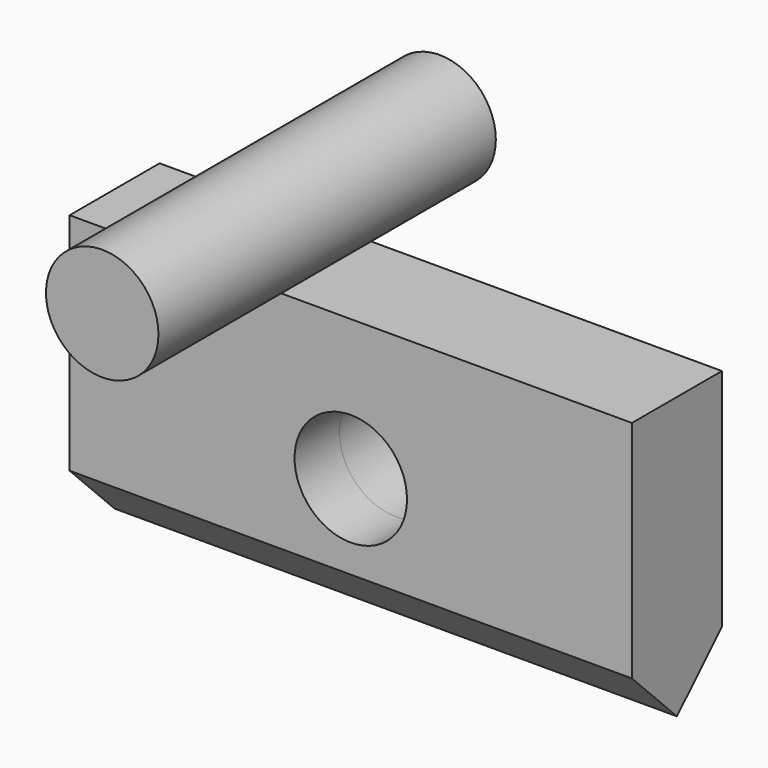
from build123d import *

# Parameters (mm, degrees)
F0_W          = 200
F0_H          = 100
F0_R          = 20
F1_DEPTH      = 20
F1_DEPTH_BACK = 20
F2_SIZE       = 19.99999
F3_R          = 20
F4_DEPTH      = 150


# Not quite as in the source:
# - a fillet or chamfer is up to 0.001 mm smaller than in the source, because OpenCascade refuses the exact size


with BuildPart() as f1:
    # F0 (on Front) → F1 (new body, two sides)
    with BuildSketch(Plane.XZ) as f1_sk:
        Rectangle(F0_W, F0_H)
        Circle(F0_R, mode=Mode.SUBTRACT)
    extrude(amount=F1_DEPTH)
    extrude(f1_sk.sketch, amount=-F1_DEPTH_BACK)

    # F2 (size 20 in the source; OpenCascade refuses exactly that, so slightly less here)
    f2_edges = [f1.edges().sort_by_distance(p)[0] for p in [
        (0, 20, -50),
        (0, -20, -50),
    ]]
    chamfer(f2_edges, length=F2_SIZE)


with BuildPart() as f4:
    # F3 (on Front) → F4 (new body)
    with BuildSketch(Plane.XZ):
        with Locations((15.5900605023, 109.6589937806)):
            Circle(F3_R)
    extrude(amount=F4_DEPTH)


solid = Compound([f1.part, f4.part])
